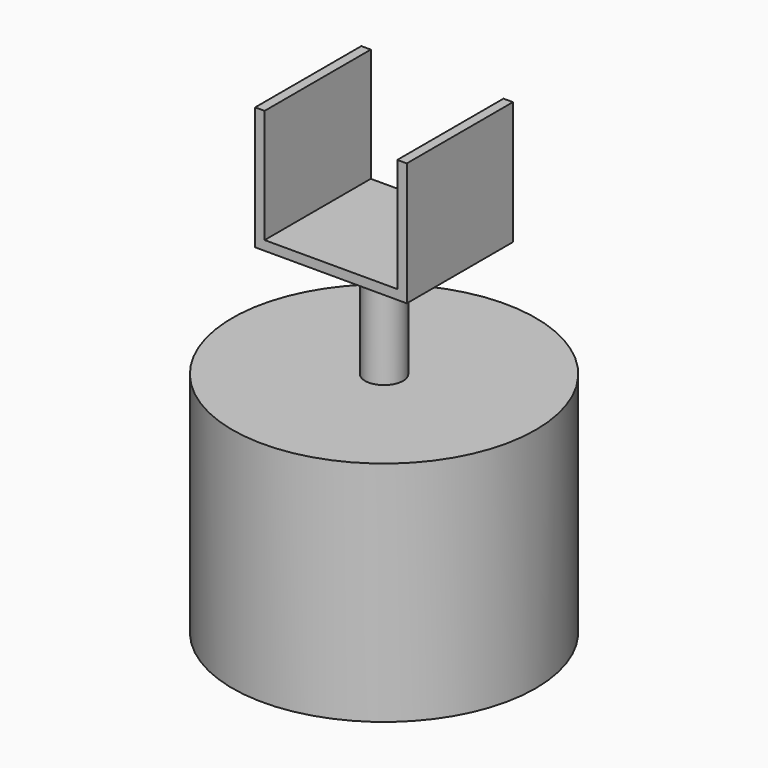
from build123d import *

# Parameters (mm, degrees)
F0_R     = 101.6
F1_DEPTH = 152.4
F2_R     = 12.7
F3_DEPTH = 76.2
F4_W     = 101.6
F4_H     = 88.9
F4_R     = 12.7
F5_DEPTH = 6.35
F6_W     = 6.35
F6_H     = 88.9
F7_DEPTH = 76.2


# Not quite as in the source:
# - a feature names something its author has since deleted; it is built from what else it names


with BuildPart() as f1:
    # F0 (on Top) → F1 (new body)
    with BuildSketch(Plane.XY):
        Circle(F0_R)
    extrude(amount=F1_DEPTH)

    # F2 (on face) → F3 (join)
    with BuildSketch(Plane.XY.offset(152.4)):
        Circle(F2_R)
    extrude(amount=F3_DEPTH)

    # F4 (on face) → F5 (join)
    with BuildSketch(Plane.XY.offset(228.6)):
        Rectangle(F4_W, F4_H)
        Circle(F4_R, mode=Mode.SUBTRACT)
        Circle(F4_R)
    extrude(amount=F5_DEPTH)

    # F6 (on face) → F7 (join)
    with BuildSketch(Plane.XY.offset(234.95)):
        with Locations((-47.625, 0)):
            Rectangle(F6_W, F6_H)
        with Locations((47.625, 0)):
            Rectangle(F6_W, F6_H)
    extrude(amount=F7_DEPTH)


solid = f1.part
